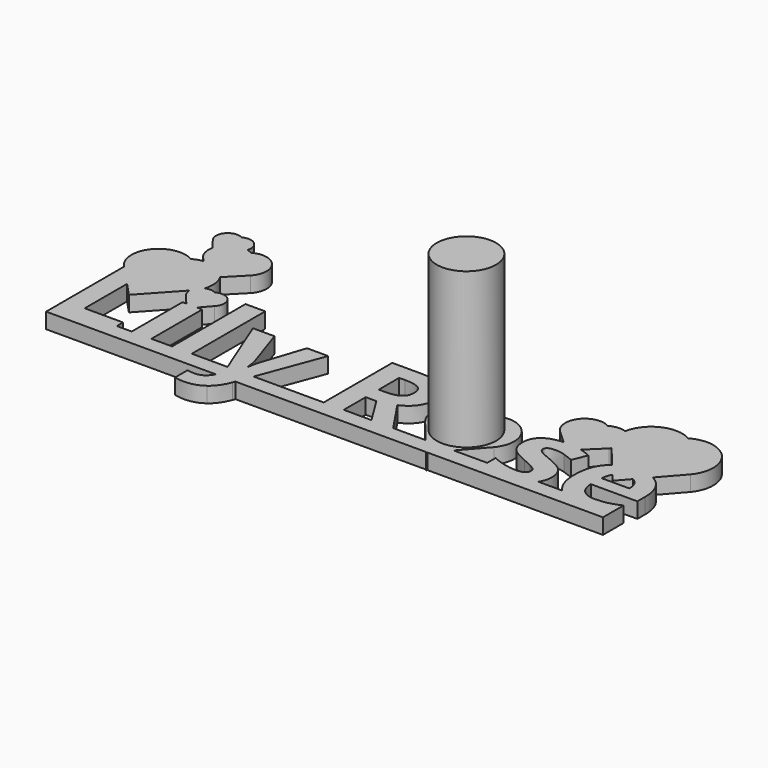
from build123d import *

# Parameters (mm, degrees)
F0_W     = 2.5421468203
F0_H     = 9.3203158344
F0_H_2   = 12.9721510883
F1_DEPTH = 2
F2_W     = 71.8336534358
F2_H     = 2
F3_DEPTH = 2
F5_DEPTH = 2
F6_R     = 3.8242127304
F7_DEPTH = 20


# Not quite as in the source:
# - a feature names something its author has since deleted; it is built from what else it names


with BuildPart() as f1:
    # F0 (on Top) → F1 (new body)
    with BuildSketch(Plane.XY):
        Polygon((-35.9661758429, -9.0986326135), (-35.9661758429, -21.2865327415), (-28.4384336321, -21.2865327415), (-28.4384336321, -19.152516523), (-33.3813486983, -19.152516523), (-33.3813486983, -9.0986326135), align=None)
        with Locations((-25.2494131455, -16.6263748243)):
            Rectangle(F0_W, F0_H)
        with Locations((-20.0397460521, -14.8004571973)):
            Rectangle(F0_W, F0_H_2)
        with BuildLine():
            Line((-14.6500213402, -11.9662169071), (-17.4349125053, -11.9662169071))
            Line((-17.4349125053, -11.9662169071), (-13.7323943662, -21.2198447347))
            Line((-13.7323943662, -21.2198447347), (-13.8844430218, -21.6786582217))
            add(Edge.make_bspline(
                [(-14.6713615023, -22.9243901892), (-14.1672001707, -22.5109245469), (-13.8844430218, -21.6786582217)],
                knots=[0, 0, 0, 1, 1, 1], degree=2))
            add(Edge.make_bspline(
                [(-15.8504054631, -23.3378558316), (-15.175522834, -23.3378558316), (-14.6713615023, -22.9243901892)],
                knots=[0, 0, 0, 1, 1, 1], degree=2))
            add(Edge.make_bspline(
                [(-16.8507255655, -23.2284875004), (-16.3919120785, -23.3378558316), (-15.8504054631, -23.3378558316)],
                knots=[0, 0, 0, 1, 1, 1], degree=2))
            Line((-16.8507255655, -23.2284875004), (-16.8507255655, -25.2451328269))
            add(Edge.make_bspline(
                [(-15.5596457533, -25.3891789216), (-16.2185232608, -25.3891789216), (-16.8507255655, -25.2451328269)],
                knots=[0, 0, 0, 1, 1, 1], degree=2))
            add(Edge.make_bspline(
                [(-13.2135616731, -24.6636134073), (-14.2178830559, -25.3891789216), (-15.5596457533, -25.3891789216)],
                knots=[0, 0, 0, 1, 1, 1], degree=2))
            add(Edge.make_bspline(
                [(-11.6650661545, -22.4789143036), (-12.2092402902, -23.938047893), (-13.2135616731, -24.6636134073)],
                knots=[0, 0, 0, 1, 1, 1], degree=2))
            Line((-11.6650661545, -22.4789143036), (-7.7224711908, -11.9662169071))
            Line((-7.7224711908, -11.9662169071), (-10.4486769099, -11.9662169071))
            Line((-10.4486769099, -11.9662169071), (-12.1745625267, -17.2105617641))
            add(Edge.make_bspline(
                [(-12.5320102433, -18.8270790497), (-12.441314554, -17.9681375217), (-12.1745625267, -17.2105617641)],
                knots=[0, 0, 0, 1, 1, 1], degree=2))
            Line((-12.5320102433, -18.8270790497), (-12.5826931285, -18.8270790497))
            add(Edge.make_bspline(
                [(-12.8921254802, -17.2105617641), (-12.6653862569, -17.8934469541), (-12.5826931285, -18.8270790497)],
                knots=[0, 0, 0, 1, 1, 1], degree=2))
            Line((-12.8921254802, -17.2105617641), (-14.6500213402, -11.9662169071))
        make_face()
        with BuildLine():
            Line((0.8322663252, -21.2865327415), (0.8322663252, -16.6103697027))
            Line((0.8322663252, -16.6103697027), (2.2060392659, -16.6103697027))
            Line((2.2060392659, -16.6103697027), (5.1163038839, -21.2865327415))
            Line((5.1163038839, -21.2865327415), (7.9838881776, -21.2865327415))
            add(Edge.make_bspline(
                [(4.3987409304, -15.9754998777), (7.1516218523, -20.0861486186), (7.9838881776, -21.2865327415)],
                knots=[0, 0, 0, 1, 1, 1], degree=2))
            add(Edge.make_bspline(
                [(6.0752774221, -14.6630799033), (5.4844216816, -15.5006812691), (4.3987409304, -15.9754998777)],
                knots=[0, 0, 0, 1, 1, 1], degree=2))
            add(Edge.make_bspline(
                [(6.6661331626, -12.7504678674), (6.6661331626, -13.8254785375), (6.0752774221, -14.6630799033)],
                knots=[0, 0, 0, 1, 1, 1], degree=2))
            add(Edge.make_bspline(
                [(5.4750853606, -10.0029219861), (6.6661331626, -10.9072113587), (6.6661331626, -12.7504678674)],
                knots=[0, 0, 0, 1, 1, 1], degree=2))
            add(Edge.make_bspline(
                [(1.7979086641, -9.0986326135), (4.2840375587, -9.0986326135), (5.4750853606, -10.0029219861)],
                knots=[0, 0, 0, 1, 1, 1], degree=2))
            Line((1.7979086641, -9.0986326135), (-1.7525608195, -9.0986326135))
            Line((-1.7525608195, -9.0986326135), (-1.7525608195, -21.2865327415))
            Line((-1.7525608195, -21.2865327415), (0.8322663252, -21.2865327415))
        make_face()
        with BuildLine():
            Line((1.6645326504, -14.5083637274), (0.8322663252, -14.5083637274))
            Line((0.8322663252, -14.5083637274), (0.8322663252, -11.2166437104))
            Line((0.8322663252, -11.2166437104), (1.6165172855, -11.2166437104))
            add(Edge.make_bspline(
                [(3.4611075544, -11.5834277479), (2.8649167734, -11.2166437104), (1.6165172855, -11.2166437104)],
                knots=[0, 0, 0, 1, 1, 1], degree=2))
            add(Edge.make_bspline(
                [(4.0572983355, -12.8171558743), (4.0572983355, -11.9502117855), (3.4611075544, -11.5834277479)],
                knots=[0, 0, 0, 1, 1, 1], degree=2))
            add(Edge.make_bspline(
                [(3.4744451558, -14.1002331256), (4.0572983355, -13.6921025239), (4.0572983355, -12.8171558743)],
                knots=[0, 0, 0, 1, 1, 1], degree=2))
            add(Edge.make_bspline(
                [(1.6645326504, -14.5083637274), (2.8915919761, -14.5083637274), (3.4744451558, -14.1002331256)],
                knots=[0, 0, 0, 1, 1, 1], degree=2))
        make_face(mode=Mode.SUBTRACT)
        with BuildLine():
            add(Edge.make_bspline(
                [(26.3924455826, -18.517646698), (26.3924455826, -19.9527726049), (25.3961267606, -20.7036795618)],
                knots=[0, 0, 0, 1, 1, 1], degree=2))
            add(Edge.make_bspline(
                [(26.1497012377, -17.326598896), (26.3924455826, -17.8267589472), (26.3924455826, -18.517646698)],
                knots=[0, 0, 0, 1, 1, 1], degree=2))
            add(Edge.make_bspline(
                [(25.3987942808, -16.4436496856), (25.9069568929, -16.8264388448), (26.1497012377, -17.326598896)],
                knots=[0, 0, 0, 1, 1, 1], degree=2))
            add(Edge.make_bspline(
                [(23.7996158771, -15.6180521611), (24.8906316688, -16.0608605264), (25.3987942808, -16.4436496856)],
                knots=[0, 0, 0, 1, 1, 1], degree=2))
            add(Edge.make_bspline(
                [(22.2097737943, -14.8764815251), (22.5725565514, -15.1272284308), (23.7996158771, -15.6180521611)],
                knots=[0, 0, 0, 1, 1, 1], degree=2))
            add(Edge.make_bspline(
                [(21.8469910371, -14.2842920245), (21.8469910371, -14.6257346195), (22.2097737943, -14.8764815251)],
                knots=[0, 0, 0, 1, 1, 1], degree=2))
            add(Edge.make_bspline(
                [(22.9726845924, -13.6760974022), (21.8469910371, -13.6760974022), (21.8469910371, -14.2842920245)],
                knots=[0, 0, 0, 1, 1, 1], degree=2))
            add(Edge.make_bspline(
                [(24.2157490397, -13.8681588619), (23.6075544174, -13.6760974022), (22.9726845924, -13.6760974022)],
                knots=[0, 0, 0, 1, 1, 1], degree=2))
            add(Edge.make_bspline(
                [(25.5255014938, -14.3589825921), (24.823943662, -14.0602203215), (24.2157490397, -13.8681588619)],
                knots=[0, 0, 0, 1, 1, 1], degree=2))
            Line((25.5255014938, -14.3589825921), (26.2910798122, -12.5263961645))
            add(Edge.make_bspline(
                [(23.0153649168, -11.7928280894), (24.6985702091, -11.7928280894), (26.2910798122, -12.5263961645)],
                knots=[0, 0, 0, 1, 1, 1], degree=2))
            add(Edge.make_bspline(
                [(20.2851579172, -12.4717119989), (21.2467989757, -11.7928280894), (23.0153649168, -11.7928280894)],
                knots=[0, 0, 0, 1, 1, 1], degree=2))
            add(Edge.make_bspline(
                [(19.3235168587, -14.3936603557), (19.3235168587, -13.1505959084), (20.2851579172, -12.4717119989)],
                knots=[0, 0, 0, 1, 1, 1], degree=2))
            add(Edge.make_bspline(
                [(19.5515898421, -15.6127171205), (19.3235168587, -15.1165583497), (19.3235168587, -14.3936603557)],
                knots=[0, 0, 0, 1, 1, 1], degree=2))
            add(Edge.make_bspline(
                [(20.2851579172, -16.4929988107), (19.7796628254, -16.1088758913), (19.5515898421, -15.6127171205)],
                knots=[0, 0, 0, 1, 1, 1], degree=2))
            add(Edge.make_bspline(
                [(21.865663679, -17.3279326562), (20.790653009, -16.87712173), (20.2851579172, -16.4929988107)],
                knots=[0, 0, 0, 1, 1, 1], degree=2))
            add(Edge.make_bspline(
                [(23.0647140418, -17.8801093527), (22.6152368758, -17.6427000484), (21.865663679, -17.3279326562)],
                knots=[0, 0, 0, 1, 1, 1], degree=2))
            add(Edge.make_bspline(
                [(23.6982501067, -18.3055788363), (23.5141912079, -18.117518657), (23.0647140418, -17.8801093527)],
                knots=[0, 0, 0, 1, 1, 1], degree=2))
            add(Edge.make_bspline(
                [(23.8823090055, -18.7950688064), (23.8823090055, -18.4936390155), (23.6982501067, -18.3055788363)],
                knots=[0, 0, 0, 1, 1, 1], degree=2))
            add(Edge.make_bspline(
                [(22.4978659838, -19.5953248883), (23.8823090055, -19.5953248883), (23.8823090055, -18.7950688064)],
                knots=[0, 0, 0, 1, 1, 1], degree=2))
            add(Edge.make_bspline(
                [(20.9346991037, -19.3699194253), (21.8229833547, -19.5953248883), (22.4978659838, -19.5953248883)],
                knots=[0, 0, 0, 1, 1, 1], degree=2))
            add(Edge.make_bspline(
                [(19.3395219804, -18.811073928), (20.0464148528, -19.1445139622), (20.9346991037, -19.3699194253)],
                knots=[0, 0, 0, 1, 1, 1], degree=2))
            Line((19.3395219804, -18.811073928), (19.3395219804, -20.910412383))
            add(Edge.make_bspline(
                [(20.6812846778, -21.3158754645), (19.9637217243, -21.1771644103), (19.3395219804, -20.910412383)],
                knots=[0, 0, 0, 1, 1, 1], degree=2))
            add(Edge.make_bspline(
                [(22.4151728553, -21.4545865187), (21.3988476312, -21.4545865187), (20.6812846778, -21.3158754645)],
                knots=[0, 0, 0, 1, 1, 1], degree=2))
            add(Edge.make_bspline(
                [(25.3961267606, -20.7036795618), (24.3998079385, -21.4545865187), (22.4151728553, -21.4545865187)],
                knots=[0, 0, 0, 1, 1, 1], degree=2))
        make_face()
        with BuildLine():
            add(Edge.make_bspline(
                [(32.5917626974, -21.4545865187), (30.3430431071, -21.4545865187), (29.0759709774, -20.2115220714)],
                knots=[0, 0, 0, 1, 1, 1], degree=2))
            add(Edge.make_bspline(
                [(34.443021767, -21.2918677821), (33.6854460094, -21.4545865187), (32.5917626974, -21.4545865187)],
                knots=[0, 0, 0, 1, 1, 1], degree=2))
            add(Edge.make_bspline(
                [(35.8674775928, -20.7957090113), (35.2005975245, -21.1291490454), (34.443021767, -21.2918677821)],
                knots=[0, 0, 0, 1, 1, 1], degree=2))
            Line((35.8674775928, -20.7957090113), (35.8674775928, -18.8270790497))
            add(Edge.make_bspline(
                [(34.3016431925, -19.3859245469), (35.0512163892, -19.211201969), (35.8674775928, -18.8270790497)],
                knots=[0, 0, 0, 1, 1, 1], degree=2))
            add(Edge.make_bspline(
                [(32.7091335894, -19.5606471248), (33.5520699957, -19.5606471248), (34.3016431925, -19.3859245469)],
                knots=[0, 0, 0, 1, 1, 1], degree=2))
            add(Edge.make_bspline(
                [(31.0259282971, -18.9524525025), (31.6261203585, -19.5606471248), (32.7091335894, -19.5606471248)],
                knots=[0, 0, 0, 1, 1, 1], degree=2))
            add(Edge.make_bspline(
                [(30.3830559112, -17.2612446493), (30.4257362356, -18.3442578802), (31.0259282971, -18.9524525025)],
                knots=[0, 0, 0, 1, 1, 1], degree=2))
            Line((30.3830559112, -17.2612446493), (36.3929790866, -17.2612446493))
            Line((36.3929790866, -17.2612446493), (36.3929790866, -16.0261827629))
            add(Edge.make_bspline(
                [(35.292626974, -12.9171878845), (36.3929790866, -14.0415476796), (36.3929790866, -16.0261827629)],
                knots=[0, 0, 0, 1, 1, 1], degree=2))
            add(Edge.make_bspline(
                [(32.2183098592, -11.7928280894), (34.1922748613, -11.7928280894), (35.292626974, -12.9171878845)],
                knots=[0, 0, 0, 1, 1, 1], degree=2))
            add(Edge.make_bspline(
                [(28.9799402475, -13.0719040603), (30.1509816475, -11.7928280894), (32.2183098592, -11.7928280894)],
                knots=[0, 0, 0, 1, 1, 1], degree=2))
            add(Edge.make_bspline(
                [(27.8088988476, -16.6930628312), (27.8088988476, -14.3509800313), (28.9799402475, -13.0719040603)],
                knots=[0, 0, 0, 1, 1, 1], degree=2))
            add(Edge.make_bspline(
                [(29.0759709774, -20.2115220714), (27.8088988476, -18.9684576242), (27.8088988476, -16.6930628312)],
                knots=[0, 0, 0, 1, 1, 1], degree=2))
        make_face()
        with BuildLine():
            add(Edge.make_bspline(
                [(32.2343149808, -13.6014068346), (31.426056338, -13.6014068346), (30.967242851, -14.113570727)],
                knots=[0, 0, 0, 1, 1, 1], degree=2))
            add(Edge.make_bspline(
                [(33.5173922322, -14.113570727), (33.0425736236, -13.6014068346), (32.2343149808, -13.6014068346)],
                knots=[0, 0, 0, 1, 1, 1], degree=2))
            add(Edge.make_bspline(
                [(34.0108834827, -15.5673692759), (33.9922108408, -14.6257346195), (33.5173922322, -14.113570727)],
                knots=[0, 0, 0, 1, 1, 1], degree=2))
            Line((34.0108834827, -15.5673692759), (30.4417413572, -15.5673692759))
            add(Edge.make_bspline(
                [(30.967242851, -14.113570727), (30.5084293641, -14.6257346195), (30.4417413572, -15.5673692759)],
                knots=[0, 0, 0, 1, 1, 1], degree=2))
        make_face(mode=Mode.SUBTRACT)
    extrude(amount=F1_DEPTH)

    # F2 (on Top) → F3 (join)
    with BuildSketch(Plane.XY):
        with Locations((-0.0493491251, -21.152516523)):
            Rectangle(F2_W, F2_H)
    extrude(amount=F3_DEPTH)

    # F4 (on Top) → F5 (join)
    with BuildSketch(Plane.XY):
        with BuildLine():
            ThreePointArc((-23.460767245, -10.5974629963), (-23.3785588051, -8.6388796142), (-25.3041368139, -8.2715154565))
            ThreePointArc((-25.3041368139, -8.2715154565), (-25.9770014142, -8.072538165), (-26.6667445679, -8.2013524302))
            ThreePointArc((-26.6667445679, -8.2013524302), (-26.8068712674, -8.5588377495), (-26.9853136504, -8.8988223982))
            Line((-26.9853136504, -8.8988223982), (-27.5531942854, -9.5173868708))
            ThreePointArc((-27.5531942854, -9.5173868708), (-27.4750741672, -10.0511126511), (-27.2132009809, -10.5226933926))
            Line((-27.2132009809, -10.5226933926), (-25.3683159452, -12.7685191303))
            Line((-25.3683159452, -12.7685191303), (-23.460767245, -10.5974629963))
        make_face()
        with BuildLine():
            ThreePointArc((-26.9853136504, -8.8988223982), (-26.8068712674, -8.5588377495), (-26.6667445679, -8.2013524302))
            ThreePointArc((-26.6667445679, -8.2013524302), (-27.2982305275, -8.7325614192), (-27.5531942854, -9.5173868708))
            Line((-27.5531942854, -9.5173868708), (-26.9853136504, -8.8988223982))
        make_face()
        with BuildLine():
            ThreePointArc((-27.5531942854, -9.5173868708), (-27.2982305275, -8.7325614192), (-26.6667445679, -8.2013524302))
            ThreePointArc((-26.6667445679, -8.2013524302), (-26.5103239544, -6.73277603), (-26.9735699478, -5.3304254314))
            Line((-26.9735699478, -5.3304254314), (-27.8705461931, -6.2434591072))
            Line((-27.8705461931, -6.2434591072), (-30.435701563, -3.633144129))
            ThreePointArc((-30.435701563, -3.633144129), (-31.1099811744, -3.7885760494), (-31.740504166, -4.0736248755))
            ThreePointArc((-31.740504166, -4.0736248755), (-36.233754687, -4.9311026842), (-36.0411839329, -9.5013854919))
            Line((-36.0411839329, -9.5013854919), (-31.7405052483, -14.0784189571))
            Line((-31.7405052483, -14.0784189571), (-27.5531942854, -9.5173868708))
        make_face()
        with BuildLine():
            ThreePointArc((-27.8705461931, -4.3197954554), (-27.3728222762, -4.7814116229), (-26.9735699478, -5.3304254314))
            Line((-26.9735699478, -5.3304254314), (-24.7982677336, -3.1161815346))
            ThreePointArc((-24.7982677336, -3.1161815346), (-24.6612476873, 0.1481262242), (-27.8705463616, 0.7604020253))
            ThreePointArc((-27.8705463616, 0.7604020253), (-28.1874425503, 0.9146740113), (-28.5228848144, 1.0228476104))
            ThreePointArc((-28.5228848144, 1.0228476104), (-28.6581354096, 0.7251189675), (-28.8546919313, 0.4637751287))
            Line((-28.8546919313, 0.4637751287), (-30.8609493077, -1.7959213583))
            Line((-30.8609493077, -1.7959213583), (-31.5607878634, -0.8613195248))
            ThreePointArc((-31.5607878634, -0.8613195248), (-31.5240164461, -2.0926519469), (-30.9036702721, -3.1569368221))
            Line((-30.9036702721, -3.1569368221), (-30.435701563, -3.633144129))
            ThreePointArc((-30.435701563, -3.633144129), (-29.0854748233, -3.7237500646), (-27.8705461931, -4.3197954554))
        make_face()
        with BuildLine():
            Line((-27.8705461931, -6.2434591072), (-26.9735699478, -5.3304254314))
            ThreePointArc((-26.9735699478, -5.3304254314), (-27.3728222762, -4.7814116229), (-27.8705461931, -4.3197954554))
            Line((-27.8705461931, -4.3197954554), (-27.8705461931, -6.2434591072))
        make_face()
        with BuildLine():
            Line((-30.435701563, -3.633144129), (-27.8705461931, -6.2434591072))
            Line((-27.8705461931, -6.2434591072), (-27.8705461931, -4.3197954554))
            ThreePointArc((-27.8705461931, -4.3197954554), (-29.0854748233, -3.7237500646), (-30.435701563, -3.633144129))
        make_face()
        with BuildLine():
            ThreePointArc((-28.8546919313, 0.4637751287), (-28.6581354096, 0.7251189675), (-28.5228848144, 1.0228476104))
            ThreePointArc((-28.5228848144, 1.0228476104), (-30.4382324156, 0.7198861396), (-31.5607878634, -0.8613195248))
            Line((-31.5607878634, -0.8613195248), (-30.8609493077, -1.7959213583))
            Line((-30.8609493077, -1.7959213583), (-28.8546919313, 0.4637751287))
        make_face()
        with BuildLine():
            ThreePointArc((-31.5607878634, -0.8613195248), (-30.4382324156, 0.7198861396), (-28.5228848144, 1.0228476104))
            ThreePointArc((-28.5228848144, 1.0228476104), (-29.002319592, 2.6549750089), (-30.6980615002, 2.7897226685))
            ThreePointArc((-30.6980615002, 2.7897226685), (-32.5699864004, 2.4863172854), (-32.6487473798, 0.5915997956))
            Line((-32.6487473798, 0.5915997956), (-31.5607878634, -0.8613195248))
        make_face()
        with BuildLine():
            ThreePointArc((17.7506930834, -17.0362158441), (17.7155922072, -12.5508427471), (13.296210027, -11.7834673264))
            ThreePointArc((13.296210027, -11.7834673264), (8.8768278469, -12.5508427471), (8.8417269707, -17.0362158441))
            Line((8.8417269707, -17.0362158441), (13.1464587205, -22.2764758987))
            Line((13.1464587205, -22.2764758987), (17.7506930834, -17.0362158441))
        make_face()
        with BuildLine():
            ThreePointArc((25.8714701993, -6.0752954382), (24.8088179916, -5.9429147282), (23.7882648545, -6.2672997795))
            ThreePointArc((23.7882648545, -6.2672997795), (20.5237176871, -6.9519580371), (20.845394908, -10.2719804622))
            Line((20.845394908, -10.2719804622), (23.8496661186, -13.0365993828))
            Line((23.8496661186, -13.0365993828), (26.9700384662, -10.0192630064))
            ThreePointArc((26.9700384662, -10.0192630064), (27.0463909251, -9.9214669404), (27.1177973635, -9.8200032077))
            Line((27.1177973635, -9.8200032077), (26.71594156, -9.3308138604))
            ThreePointArc((26.71594156, -9.3308138604), (25.9349212346, -7.7961222711), (25.8714701993, -6.0752954382))
        make_face()
        with BuildLine():
            ThreePointArc((31.8067793387, -3.3276726974), (28.1263885962, -3.1618587554), (25.8714701993, -6.0752954382))
            ThreePointArc((25.8714701993, -6.0752954382), (27.4103355788, -7.6428821436), (27.1177973635, -9.8200032077))
            Line((27.1177973635, -9.8200032077), (31.6356349884, -15.3196824942))
            Line((31.6356349884, -15.3196824942), (36.8976171174, -9.3308138604))
            ThreePointArc((36.8976171174, -9.3308138604), (36.8575018303, -4.2046731782), (31.8067793387, -3.3276726974))
        make_face()
        with BuildLine():
            ThreePointArc((27.1177973635, -9.8200032077), (27.4103355788, -7.6428821436), (25.8714701993, -6.0752954382))
            ThreePointArc((25.8714701993, -6.0752954382), (25.9349212346, -7.7961222711), (26.71594156, -9.3308138604))
            Line((26.71594156, -9.3308138604), (27.1177973635, -9.8200032077))
        make_face()
        with BuildLine():
            ThreePointArc((10.0142014591, -9.0243846608), (9.9891294046, -5.8205467344), (6.8324278474, -5.2724214339))
            ThreePointArc((6.8324278474, -5.2724214339), (3.6757262901, -5.8205467344), (3.6506542357, -9.0243846608))
            Line((3.6506542357, -9.0243846608), (6.7254626285, -12.7674275569))
            Line((6.7254626285, -12.7674275569), (10.0142014591, -9.0243846608))
        make_face()
    extrude(amount=F5_DEPTH)

    # F6 (on face) → F7 (join)
    with BuildSketch(Plane.XY.offset(2)):
        with Locations((13.2179185748, -15.8536620438)):
            Circle(F6_R)
    extrude(amount=F7_DEPTH)


solid = f1.part
